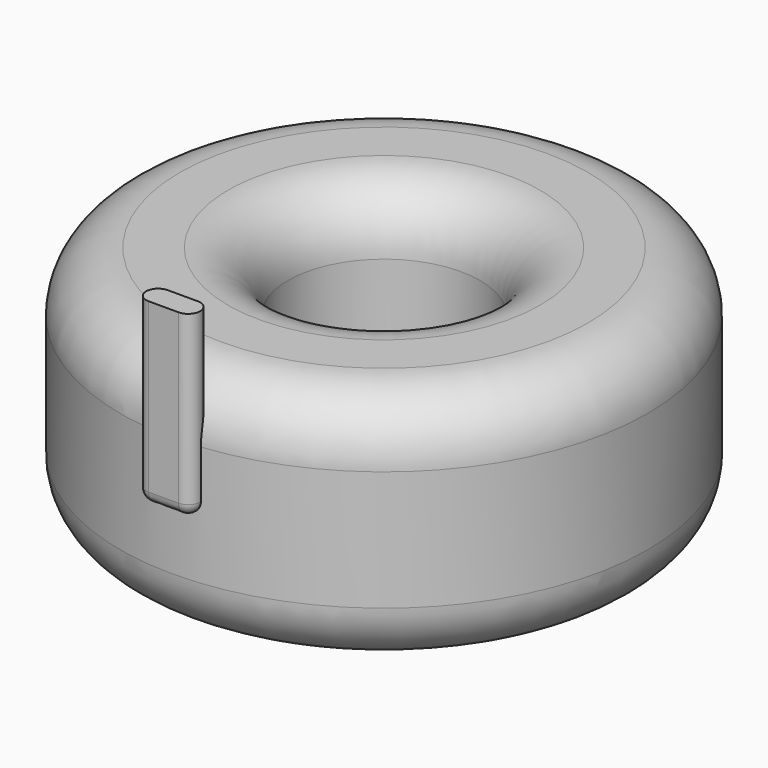
from build123d import *

# Parameters (mm, degrees)
F0_R     = 44
F0_R_2   = 16
F1_DEPTH = 20
F2_R     = 10
F4_DEPTH = 30
F5_R     = 1.9999


# Not quite as in the source:
# - a fillet or chamfer is up to 0.001 mm smaller than in the source, because OpenCascade refuses the exact size


with BuildPart() as f1:
    # F0 (on Top) → F1 (new body, symmetric)
    with BuildSketch(Plane.XY):
        Circle(F0_R)
        Circle(F0_R_2, mode=Mode.SUBTRACT)
    extrude(amount=F1_DEPTH, both=True)

    # F2
    f2_edges = [f1.edges().sort_by_distance(p)[0] for p in [
        (-16, 0, 20),
        (16, 0, 0),
        (-16, 0, -20),
        (-44, 0, -20),
        (44, 0, 0),
        (-44, 0, 20),
    ]]
    fillet(f2_edges, radius=F2_R)

    # F3 (on Top) → F4 (join)
    with BuildSketch(Plane.XY):
        with BuildLine():
            Line((2.5, -41.9289198592), (-2.5, -41.9289198592))
            ThreePointArc((-2.5, -41.9289198592), (-4.5, -43.9289198592), (-2.5, -45.9289198592))
            Line((-2.5, -45.9289198592), (2.5, -45.9289198592))
            ThreePointArc((2.5, -45.9289198592), (4.5, -43.9289198592), (2.5, -41.9289198592))
        make_face()
    extrude(amount=F4_DEPTH)

    # F5 (radius 2 in the source; OpenCascade refuses exactly that, so slightly less here)
    f5_edges = [f1.edges().sort_by_distance(p)[0] for p in [
        (0, -45.92892, 0),
    ]]
    fillet(f5_edges, radius=F5_R)


solid = f1.part
